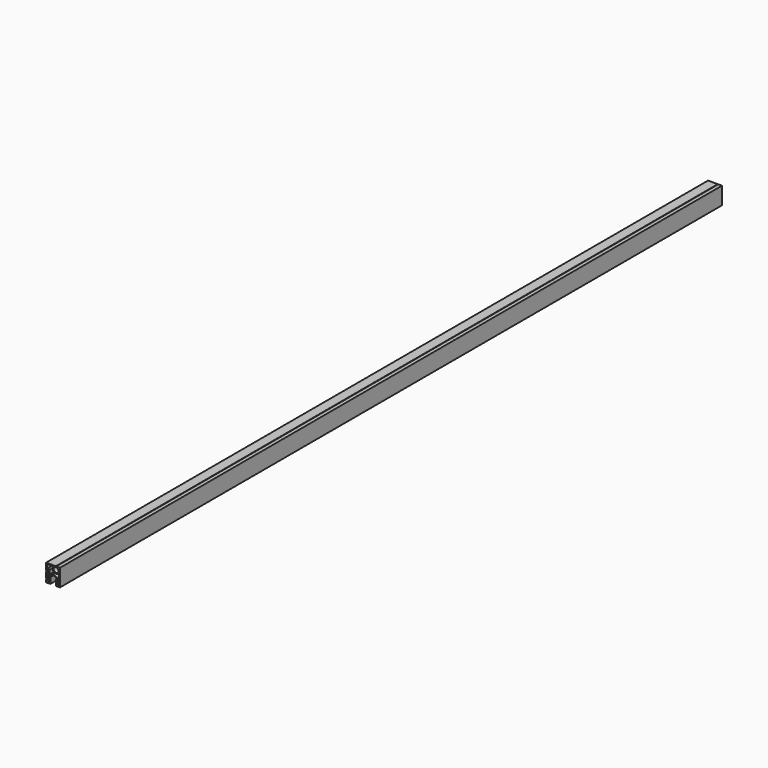
from build123d import *

# Parameters (mm, degrees)
F2_DEPTH = 1910


# Not quite as in the source:
# - a feature of the source that left no trace in its solid (it failed there, or was rolled back) is left out


with BuildPart() as f2:
    # F1 (on Front) → F2 (new body)
    with BuildSketch(Plane.XZ):
        with BuildLine():
            Line((7.5, 37.974085065), (7.5, 40))
            Line((7.5, 40), (-15, 40))
            Line((-15, 40), (-15, 37))
            Line((-15, 37), (-15, 31))
            Line((-15, 31), (-15, 29))
            Line((-15, 29), (-15, 26))
            Line((-15, 26), (-15, 24))
            Line((-15, 24), (-13, 24))
            Line((-13, 24), (-11, 24))
            Line((-11, 24), (-11, 26))
            Line((-11, 26), (-9, 26))
            Line((-9, 26), (-9, 20))
            Line((-9, 20), (-11, 20))
            Line((-11, 20), (-11, 22))
            Line((-11, 22), (-15, 22))
            Line((-15, 22), (-15, 18))
            Line((-15, 18), (-15, 7.7))
            Line((-15, 7.7), (-13, 7.7))
            Line((-13, 7.7), (-13, 11.4920835048))
            Line((-13, 11.4920835048), (-7, 11.4920835048))
            Line((-7, 11.4920835048), (-7, 3.7))
            Line((-7, 3.7), (-11, 3.7))
            Line((-11, 3.7), (-11, 5.7))
            Line((-11, 5.7), (-15, 5.7))
            Line((-15, 5.7), (-15, 3))
            Line((-15, 3), (-15, 0))
            Line((-15, 0), (-13, 0))
            Line((-13, 0), (-12, 0))
            Line((-12, 0), (-5, 0))
            Line((-5, 0), (-5, 13.4920835048))
            Line((-5, 13.4920835048), (-7, 13.4920835048))
            Line((-7, 13.4920835048), (-9.1588944197, 13.4920835048))
            Line((-9.1588944197, 13.4920835048), (-9.1588944197, 15.4920835048))
            Line((-9.1588944197, 15.4920835048), (1.5, 20))
            Line((1.5, 20), (10.8411055803, 15.4920835048))
            Line((10.8411055803, 15.4920835048), (10.8411055803, 13.4920835048))
            Line((10.8411055803, 13.4920835048), (8, 13.4920835048))
            Line((8, 13.4920835048), (8, 0))
            Line((8, 0), (17, 0))
            Line((17, 0), (17, 40))
            Line((17, 40), (8.5, 40))
            Line((8.5, 40), (8.5, 37.974085065))
            ThreePointArc((8.5, 37.974085065), (11.5604089792, 36.6859489396), (13.3185590744, 33.8691589154))
            Line((13.3185590744, 33.8691589154), (13.4318527537, 31.7073867348))
            ThreePointArc((13.4318527537, 31.7073867348), (4.0126863822, 28.7323088758), (7.5, 37.974085065))
        make_face()
        Polygon((-8.3634709733, 18), (-11.1588944197, 16.817744602), (-11.1588944197, 15.4920835048), (-11.1588944197, 13.4920835048), (-13, 13.4920835048), (-13, 18), align=None, mode=Mode.SUBTRACT)
        with BuildLine():
            Line((-13, 34), (-13, 37.9999987781))
            Line((-13, 37.9999987781), (2.9081163149, 37.9999987781))
            ThreePointArc((2.9081163149, 37.9999987781), (3.810445381, 26.2974906682), (15, 29.8410427327))
            Line((15, 29.8410427327), (15, 2))
            Line((15, 2), (10, 2))
            Line((10, 2), (10, 12))
            Line((10, 12), (12.8411055803, 12))
            Line((12.8411055803, 12), (12.8411055803, 16.7476188273))
            Line((12.8411055803, 16.7476188273), (1.5543358685, 22.194491783))
            Line((1.5543358685, 22.194491783), (-7, 18.5766464184))
            Line((-7, 18.5766464184), (-7, 28))
            Line((-7, 28), (-13, 28))
            Line((-13, 28), (-13, 34))
        make_face(mode=Mode.SUBTRACT)
        with BuildLine():
            Line((13.0918836851, 37.9999987781), (13.1020709306, 37.9999987781))
            Line((13.1020709306, 37.9999987781), (13.1025921338, 37.9900536295))
            ThreePointArc((13.1025921338, 37.9900536295), (13.0972403349, 37.9950288154), (13.0918836851, 37.9999987781))
        make_face(mode=Mode.SUBTRACT)
    extrude(amount=-F2_DEPTH)


solid = f2.part
